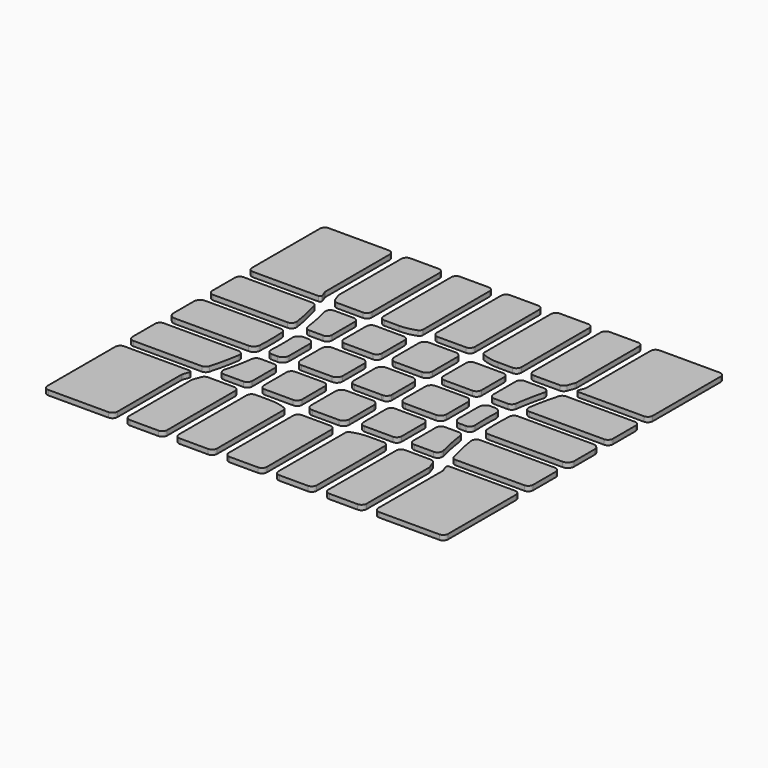
from build123d import *

# Parameters (mm, degrees)
F1_DEPTH = 1


with BuildPart() as f1:
    # F0 (on Top) → F1 (new body)
    with BuildSketch(Plane.XY):
        with BuildLine():
            Line((-41, -17.5), (-41, -34.85))
            ThreePointArc((-41, -34.85), (-40.7071067812, -35.5571067812), (-40, -35.85))
            Line((-40, -35.85), (-27.7, -35.85))
            ThreePointArc((-27.7, -35.85), (-26.9928932188, -35.5571067812), (-26.7, -34.85))
            Line((-26.7, -34.85), (-26.7, -18.4621233882))
            ThreePointArc((-26.7, -18.4621233882), (-26.6825005234, -18.2758635653), (-26.6306145568, -18.0961226413))
            ThreePointArc((-26.6306145568, -18.0961226413), (-26.426443868, -17.5681321276), (-26.2283316424, -17.0378386251))
            ThreePointArc((-26.2283316424, -17.0378386251), (-26.9318071828, -17.1289809489), (-26.6038319932, -16.5))
            Line((-26.6038319932, -16.5), (-26.7, -16.5))
            Line((-26.7, -16.5), (-40, -16.5))
            ThreePointArc((-40, -16.5), (-40.7071067812, -16.7928932188), (-41, -17.5))
        make_face()
        with BuildLine():
            ThreePointArc((-26.2038319932, -16.9), (-26.3209892807, -16.6171572875), (-26.6038319932, -16.5))
            ThreePointArc((-26.6038319932, -16.5), (-26.9318071828, -17.1289809489), (-26.2283316424, -17.0378386251))
            ThreePointArc((-26.2283316424, -17.0378386251), (-26.2100045307, -16.9699994989), (-26.2038319932, -16.9))
        make_face()
    extrude(amount=F1_DEPTH)


with BuildPart() as f1b:
    # F0 (on Top) → F1, piece 2 (new body)
    with BuildSketch(Plane.XY):
        with BuildLine():
            ThreePointArc((-26.0048854013, -14.1), (-25.4009076304, -13.897001162), (-25.0421434308, -13.3704217045))
            ThreePointArc((-25.0421434308, -13.3704217045), (-24.3126554737, -10.4301356206), (-23.7646074186, -7.4506930109))
            ThreePointArc((-23.7646074186, -7.4506930109), (-23.9946720366, -6.6483455712), (-24.7531880256, -6.3))
            Line((-24.7531880256, -6.3), (-40, -6.3))
            ThreePointArc((-40, -6.3), (-40.7071067812, -6.5928932188), (-41, -7.3))
            Line((-41, -7.3), (-41, -13.1))
            ThreePointArc((-41, -13.1), (-40.7071067812, -13.8071067812), (-40, -14.1))
            Line((-40, -14.1), (-26.0048854013, -14.1))
        make_face()
    extrude(amount=F1_DEPTH)


with BuildPart() as f1c:
    # F0 (on Top) → F1, piece 3 (new body)
    with BuildSketch(Plane.XY):
        with BuildLine():
            ThreePointArc((-23.7254457916, -17.1688294134), (-23.9746793424, -17.8630990122), (-24.2337658827, -18.5537521838))
            ThreePointArc((-24.2337658827, -18.5537521838), (-24.2833020601, -18.7296556999), (-24.3, -18.9116366293))
            Line((-24.3, -18.9116366293), (-24.3, -34.85))
            ThreePointArc((-24.3, -34.85), (-24.0071067812, -35.5571067812), (-23.3, -35.85))
            Line((-23.3, -35.85), (-17.5, -35.85))
            ThreePointArc((-17.5, -35.85), (-16.7928932188, -35.5571067812), (-16.5, -34.85))
            Line((-16.5, -34.85), (-16.5, -17.5))
            ThreePointArc((-16.5, -17.5), (-16.7928932188, -16.7928932188), (-17.5, -16.5))
            Line((-17.5, -16.5), (-22.781874892, -16.5))
            ThreePointArc((-22.781874892, -16.5), (-23.3601608997, -16.6841658911), (-23.7254457916, -17.1688294134))
        make_face()
    extrude(amount=F1_DEPTH)


with BuildPart() as f1d:
    # F0 (on Top) → F1, piece 4 (new body)
    with BuildSketch(Plane.XY):
        with BuildLine():
            ThreePointArc((-21.2970717651, -7.1618545553), (-21.7780559628, -10.0226661945), (-22.4183065056, -12.8520951609))
            ThreePointArc((-22.4183065056, -12.8520951609), (-22.2394287066, -13.713227185), (-21.4495221175, -14.1))
            Line((-21.4495221175, -14.1), (-17.5, -14.1))
            ThreePointArc((-17.5, -14.1), (-16.7928932188, -13.8071067812), (-16.5, -13.1))
            Line((-16.5, -13.1), (-16.5, -7.3))
            ThreePointArc((-16.5, -7.3), (-16.7928932188, -6.5928932188), (-17.5, -6.3))
            Line((-17.5, -6.3), (-20.3066598123, -6.3))
            ThreePointArc((-20.3066598123, -6.3), (-20.9631103266, -6.5456309111), (-21.2970717651, -7.1618545553))
        make_face()
    extrude(amount=F1_DEPTH)


with BuildPart() as f1e:
    # F0 (on Top) → F1, piece 5 (new body)
    with BuildSketch(Plane.XY):
        with BuildLine():
            ThreePointArc((-14.1, -34.85), (-13.8071067812, -35.5571067812), (-13.1, -35.85))
            Line((-13.1, -35.85), (-7.3, -35.85))
            ThreePointArc((-7.3, -35.85), (-6.5928932188, -35.5571067812), (-6.3, -34.85))
            Line((-6.3, -34.85), (-6.3, -17.8070289129))
            ThreePointArc((-6.3, -17.8070289129), (-6.4191329646, -17.4163967494), (-6.735981392, -17.1587279222))
            ThreePointArc((-6.735981392, -17.1587279222), (-8.3860466991, -16.6662310555), (-10.1, -16.5))
            Line((-10.1, -16.5), (-13.1, -16.5))
            ThreePointArc((-13.1, -16.5), (-13.8071067812, -16.7928932188), (-14.1, -17.5))
            Line((-14.1, -17.5), (-14.1, -34.85))
        make_face()
    extrude(amount=F1_DEPTH)


with BuildPart() as f1f:
    # F0 (on Top) → F1, piece 6 (new body)
    with BuildSketch(Plane.XY):
        with BuildLine():
            Line((2.9, -17.35), (-2.9, -17.35))
            ThreePointArc((-2.9, -17.35), (-3.6071067812, -17.6428932188), (-3.9, -18.35))
            Line((-3.9, -18.35), (-3.9, -34.85))
            ThreePointArc((-3.9, -34.85), (-3.6071067812, -35.5571067812), (-2.9, -35.85))
            Line((-2.9, -35.85), (2.9, -35.85))
            ThreePointArc((2.9, -35.85), (3.6071067812, -35.5571067812), (3.9, -34.85))
            Line((3.9, -34.85), (3.9, -18.35))
            ThreePointArc((3.9, -18.35), (3.6071067812, -17.6428932188), (2.9, -17.35))
        make_face()
    extrude(amount=F1_DEPTH)


with BuildPart() as f1g:
    # F0 (on Top) → F1, piece 7 (new body)
    with BuildSketch(Plane.XY):
        with BuildLine():
            ThreePointArc((-24.5702589826, -3.9), (-23.6761868462, -3.5437346104), (-23.2721561836, -2.6702077151))
            ThreePointArc((-23.2721561836, -2.6702077151), (-23.2002128063, 0.1450636286), (-23.2886746909, 2.9598643468))
            ThreePointArc((-23.2886746909, 2.9598643468), (-23.6012662868, 3.6279644039), (-24.2868812126, 3.9))
            Line((-24.2868812126, 3.9), (-39.7, 3.9))
            ThreePointArc((-39.7, 3.9), (-40.6192388155, 3.5192388155), (-41, 2.6))
            Line((-41, 2.6), (-41, -2.6))
            ThreePointArc((-41, -2.6), (-40.6192388155, -3.5192388155), (-39.7, -3.9))
            Line((-39.7, -3.9), (-24.5702589826, -3.9))
        make_face()
    extrude(amount=F1_DEPTH)


with BuildPart() as f1h:
    # F0 (on Top) → F1, piece 8 (new body)
    with BuildSketch(Plane.XY):
        with BuildLine():
            ThreePointArc((-20.8620834649, 2.5363978495), (-20.8002304252, -0.1545695617), (-20.8781285413, -2.8451203028))
            ThreePointArc((-20.8781285413, -2.8451203028), (-20.6058861086, -3.5874301066), (-19.8796355674, -3.9))
            Line((-19.8796355674, -3.9), (-18.65, -3.9))
            ThreePointArc((-18.65, -3.9), (-17.7307611845, -3.5192388155), (-17.35, -2.6))
            Line((-17.35, -2.6), (-17.35, 2.6))
            ThreePointArc((-17.35, 2.6), (-17.7307611845, 3.5192388155), (-18.65, 3.9))
            Line((-18.65, 3.9), (-19.5636402561, 3.9))
            ThreePointArc((-19.5636402561, 3.9), (-20.5050973172, 3.4964700788), (-20.8620834649, 2.5363978495))
        make_face()
    extrude(amount=F1_DEPTH)


with BuildPart() as f1i:
    # F0 (on Top) → F1, piece 9 (new body)
    with BuildSketch(Plane.XY):
        with BuildLine():
            Line((-7.3, -6.3), (-13.1, -6.3))
            ThreePointArc((-13.1, -6.3), (-13.8071067812, -6.5928932188), (-14.1, -7.3))
            Line((-14.1, -7.3), (-14.1, -13.1))
            ThreePointArc((-14.1, -13.1), (-13.8071067812, -13.8071067812), (-13.1, -14.1))
            Line((-13.1, -14.1), (-7.3, -14.1))
            ThreePointArc((-7.3, -14.1), (-6.5928932188, -13.8071067812), (-6.3, -13.1))
            Line((-6.3, -13.1), (-6.3, -7.3))
            ThreePointArc((-6.3, -7.3), (-6.5928932188, -6.5928932188), (-7.3, -6.3))
        make_face()
    extrude(amount=F1_DEPTH)


with BuildPart() as f1j:
    # F0 (on Top) → F1, piece 10 (new body)
    with BuildSketch(Plane.XY):
        with BuildLine():
            Line((2.7, -6.3), (-2.7, -6.3))
            ThreePointArc((-2.7, -6.3), (-3.5485281374, -6.6514718626), (-3.9, -7.5))
            Line((-3.9, -7.5), (-3.9, -13.75))
            ThreePointArc((-3.9, -13.75), (-3.5485281374, -14.5985281374), (-2.7, -14.95))
            Line((-2.7, -14.95), (2.7, -14.95))
            ThreePointArc((2.7, -14.95), (3.5485281374, -14.5985281374), (3.9, -13.75))
            Line((3.9, -13.75), (3.9, -7.5))
            ThreePointArc((3.9, -7.5), (3.5485281374, -6.6514718626), (2.7, -6.3))
        make_face()
    extrude(amount=F1_DEPTH)


with BuildPart() as f1k:
    # F0 (on Top) → F1, piece 11 (new body)
    with BuildSketch(Plane.XY):
        with BuildLine():
            Line((2.6, 3.9), (-2.6, 3.9))
            ThreePointArc((-2.6, 3.9), (-3.5192388155, 3.5192388155), (-3.9, 2.6))
            Line((-3.9, 2.6), (-3.9, -2.6))
            ThreePointArc((-3.9, -2.6), (-3.5192388155, -3.5192388155), (-2.6, -3.9))
            Line((-2.6, -3.9), (2.9, -3.9))
            ThreePointArc((2.9, -3.9), (3.6071067812, -3.6071067812), (3.9, -2.9))
            Line((3.9, -2.9), (3.9, 2.6))
            ThreePointArc((3.9, 2.6), (3.5192388155, 3.5192388155), (2.6, 3.9))
        make_face()
    extrude(amount=F1_DEPTH)


with BuildPart() as f1l:
    # F0 (on Top) → F1, piece 12 (new body)
    with BuildSketch(Plane.XY):
        with BuildLine():
            ThreePointArc((-6.3, 2.7), (-6.6514718626, 3.5485281374), (-7.5, 3.9))
            Line((-7.5, 3.9), (-13.75, 3.9))
            ThreePointArc((-13.75, 3.9), (-14.5985281374, 3.5485281374), (-14.95, 2.7))
            Line((-14.95, 2.7), (-14.95, -2.7))
            ThreePointArc((-14.95, -2.7), (-14.5985281374, -3.5485281374), (-13.75, -3.9))
            Line((-13.75, -3.9), (-7.5, -3.9))
            ThreePointArc((-7.5, -3.9), (-6.6514718626, -3.5485281374), (-6.3, -2.7))
            Line((-6.3, -2.7), (-6.3, 2.7))
        make_face()
    extrude(amount=F1_DEPTH)


with BuildPart() as f2_1:
    # F2: instance of F1
    add(f1.part.mirror(Plane.XZ))


with BuildPart() as f2_2:
    # F2: instance of F1b
    add(f1b.part.mirror(Plane.XZ))


with BuildPart() as f2_3:
    # F2: instance of F1c
    add(f1c.part.mirror(Plane.XZ))


with BuildPart() as f2_4:
    # F2: instance of F1d
    add(f1d.part.mirror(Plane.XZ))


with BuildPart() as f2_5:
    # F2: instance of F1e
    add(f1e.part.mirror(Plane.XZ))


with BuildPart() as f2_6:
    # F2: instance of F1f
    add(f1f.part.mirror(Plane.XZ))


with BuildPart() as f2_7:
    # F2: instance of F1i
    add(f1i.part.mirror(Plane.XZ))


with BuildPart() as f2_8:
    # F2: instance of F1j
    add(f1j.part.mirror(Plane.XZ))


with BuildPart() as f3_1:
    # F3: instance of F2_1
    add(f2_1.part.mirror(Plane.YZ))


with BuildPart() as f3_2:
    # F3: instance of F2_2
    add(f2_2.part.mirror(Plane.YZ))


with BuildPart() as f3_3:
    # F3: instance of F1g
    add(f1g.part.mirror(Plane.YZ))


with BuildPart() as f3_4:
    # F3: instance of F1b
    add(f1b.part.mirror(Plane.YZ))


with BuildPart() as f3_5:
    # F3: instance of F1
    add(f1.part.mirror(Plane.YZ))


with BuildPart() as f3_6:
    # F3: instance of F1c
    add(f1c.part.mirror(Plane.YZ))


with BuildPart() as f3_7:
    # F3: instance of F1d
    add(f1d.part.mirror(Plane.YZ))


with BuildPart() as f3_8:
    # F3: instance of F1h
    add(f1h.part.mirror(Plane.YZ))


with BuildPart() as f3_9:
    # F3: instance of F2_4
    add(f2_4.part.mirror(Plane.YZ))


with BuildPart() as f3_10:
    # F3: instance of F2_3
    add(f2_3.part.mirror(Plane.YZ))


with BuildPart() as f3_11:
    # F3: instance of F2_5
    add(f2_5.part.mirror(Plane.YZ))


with BuildPart() as f3_12:
    # F3: instance of F2_7
    add(f2_7.part.mirror(Plane.YZ))


with BuildPart() as f3_13:
    # F3: instance of F1l
    add(f1l.part.mirror(Plane.YZ))


with BuildPart() as f3_14:
    # F3: instance of F1i
    add(f1i.part.mirror(Plane.YZ))


with BuildPart() as f3_15:
    # F3: instance of F1e
    add(f1e.part.mirror(Plane.YZ))


with BuildPart() as f3_16:
    # F3: instance of F1f
    add(f1f.part.mirror(Plane.YZ))


with BuildPart() as f3_17:
    # F3: instance of F1j
    add(f1j.part.mirror(Plane.YZ))


with BuildPart() as f3_18:
    # F3: instance of F1k
    add(f1k.part.mirror(Plane.YZ))


with BuildPart() as f3_19:
    # F3: instance of F2_8
    add(f2_8.part.mirror(Plane.YZ))


with BuildPart() as f3_20:
    # F3: instance of F2_6
    add(f2_6.part.mirror(Plane.YZ))


solid = Compound([f1.part, f1b.part, f1c.part, f1d.part, f1e.part, f1f.part, f1g.part, f1h.part, f1i.part, f1j.part, f1k.part, f1l.part, f2_1.part, f2_2.part, f2_3.part, f2_4.part, f2_5.part, f2_6.part, f2_7.part, f2_8.part, f3_1.part, f3_2.part, f3_3.part, f3_4.part, f3_5.part, f3_6.part, f3_7.part, f3_8.part, f3_9.part, f3_10.part, f3_11.part, f3_12.part, f3_13.part, f3_14.part, f3_15.part, f3_16.part, f3_17.part, f3_18.part, f3_19.part, f3_20.part])
